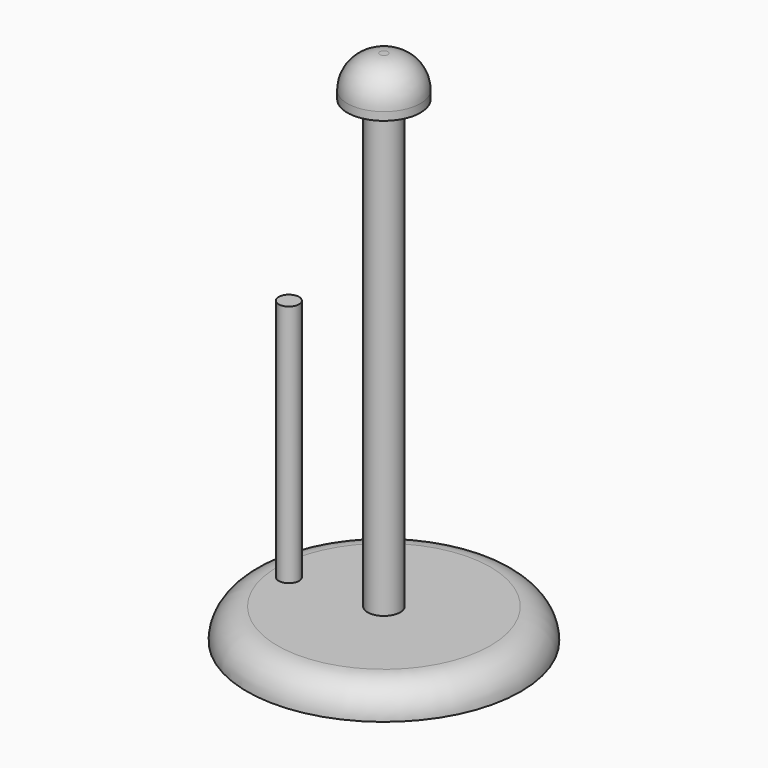
from build123d import *

# Parameters (mm, degrees)
F0_R     = 85.725
F1_DEPTH = 19.05
F2_R     = 19.04999
F3_R     = 10.16
F4_DEPTH = 279.4
F5_R     = 22.86
F6_DEPTH = 25.4
F7_R     = 20.32
F8_R     = 6.35
F9_DEPTH = 152.4


# Not quite as in the source:
# - a fillet or chamfer is up to 0.001 mm smaller than in the source, because OpenCascade refuses the exact size


with BuildPart() as f1:
    # F0 (on Top) → F1 (new body)
    with BuildSketch(Plane.XY):
        Circle(F0_R)
    extrude(amount=F1_DEPTH)

    # F2 (radius 19.05 in the source; OpenCascade refuses exactly that, so slightly less here)
    f2_edges = [f1.edges().sort_by_distance(p)[0] for p in [
        (-85.725, 0, 19.05),
    ]]
    fillet(f2_edges, radius=F2_R)

    # F3 (on face) → F4 (join)
    with BuildSketch(Plane.XY.offset(19.05)):
        Circle(F3_R)
    extrude(amount=F4_DEPTH)

    # F5 (on face) → F6 (join)
    with BuildSketch(Plane.XY.offset(298.45)):
        Circle(F5_R)
    extrude(amount=F6_DEPTH)

    # F7
    f7_edges = [f1.edges().sort_by_distance(p)[0] for p in [
        (-22.86, 0, 323.85),
    ]]
    fillet(f7_edges, radius=F7_R)

    # F8 (on face) → F9 (join)
    with BuildSketch(Plane.XY.offset(19.05)):
        with Locations((-55.5577278137, -4.9048527144)):
            Circle(F8_R)
    extrude(amount=F9_DEPTH)


solid = f1.part
